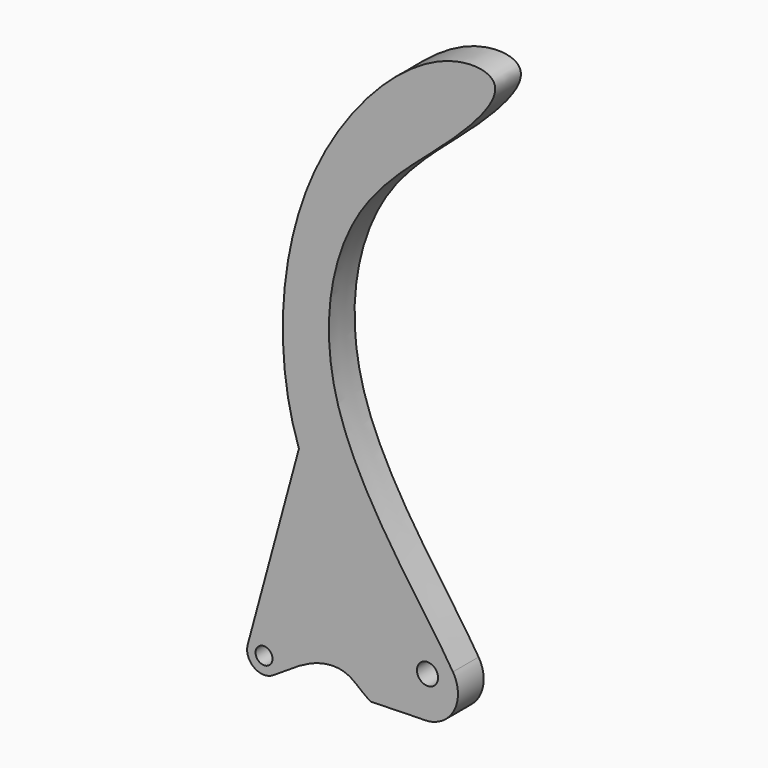
from build123d import *

# Parameters (mm, degrees)
F0_R     = 1.27
F0_R_2   = 1.5875
F1_DEPTH = 4.826
F2_R     = 5.08


with BuildPart() as f1:
    # F0 (on Front) → F1 (new body)
    with BuildSketch(Plane.XZ):
        with BuildLine():
            add(Edge.make_bspline(
                [(-5.7409273062, -27.357215091), (-3.6683374093, -26.0328951082), (-0.0251701264, -23.2850982777), (5.6115406498, -22.8429500303), (7.6257882882, -25.3641492448), (8.9509775862, -26.0758455843)],
                knots=[0, 0, 0, 0, 0.3817939574, 0.6994189819, 1, 1, 1, 1], degree=3))
            Line((8.9509775862, -26.0758455843), (16.1743344595, -25.8907967367))
            add(Edge.make_bspline(
                [(16.1743344595, -25.8907967367), (14.5463270907, -22.5263236355), (12.9183197219, -19.1618505343), (10.2751832414, -15.4096915571)],
                knots=[0, 0, 0, 0, 0.077888926, 0.077888926, 0.077888926, 0.077888926], degree=3))
            add(Edge.make_bspline(
                [(10.2751832414, -15.4096915571), (6.6364516561, -10.2441999209), (1.0738216148, -4.3439561733), (-1.8614867632, 3.8848498313)],
                knots=[0.077888926, 0.077888926, 0.077888926, 0.077888926, 0.1851164178, 0.1851164178, 0.1851164178, 0.1851164178], degree=3))
            Line((-1.8614867632, 3.8848498313), (-9.560300399, -24.553100254))
            ThreePointArc((-9.560300399, -24.553100254), (-6.7737644216, -22.6990049585), (-4.5685573119, -25.216844056))
            ThreePointArc((-4.5685573119, -25.216844056), (-4.8808477017, -26.4370530106), (-5.7409273062, -27.357215091))
        make_face()
        with BuildLine():
            ThreePointArc((-9.560300399, -24.553100254), (-8.6117506787, -27.264283848), (-5.7409273062, -27.357215091))
            ThreePointArc((-5.7409273062, -27.357215091), (-4.8808477017, -26.4370530106), (-4.5685573119, -25.216844056))
            ThreePointArc((-4.5685573119, -25.216844056), (-6.7737644216, -22.6990049585), (-9.560300399, -24.553100254))
        make_face()
        with Locations((-7.1085573119, -25.216844056)):
            Circle(F0_R, mode=Mode.SUBTRACT)
        with BuildLine():
            add(Edge.make_bspline(
                [(16.1743344595, -25.8907967367), (14.5463270907, -22.5263236355), (12.9183197219, -19.1618505343), (10.2751832414, -15.4096915571)],
                knots=[0, 0, 0, 0, 0.077888926, 0.077888926, 0.077888926, 0.077888926], degree=3))
            Line((16.1743344595, -25.8907967367), (25.5930349231, -25.8907967367))
            add(Edge.make_bspline(
                [(-1.8614867632, 3.8848498313), (-5.5713200583, 14.284949093), (-4.6432671747, 41.195895922), (17.1641890949, 64.2564894171), (30.9795358991, 62.8017285805), (20.3263989801, 50.5876190519), (4.3365893948, 39.2173794204), (-0.4864534789, 10.7428135064), (19.8393789476, -14.7354313612), (23.9996070336, -22.8014096788), (25.5930349231, -25.8907967367)],
                knots=[0.1851164178, 0.1851164178, 0.1851164178, 0.1851164178, 0.3206374834, 0.4434091583, 0.50463888, 0.5800628175, 0.6816083979, 0.7958783822, 0.9218184504, 1, 1, 1, 1], degree=3))
            add(Edge.make_bspline(
                [(10.2751832414, -15.4096915571), (6.6364516561, -10.2441999209), (1.0738216148, -4.3439561733), (-1.8614867632, 3.8848498313)],
                knots=[0.077888926, 0.077888926, 0.077888926, 0.077888926, 0.1851164178, 0.1851164178, 0.1851164178, 0.1851164178], degree=3))
        make_face()
        with Locations((17.4575652927, -19.6446664631)):
            Circle(F0_R_2, mode=Mode.SUBTRACT)
    extrude(amount=F1_DEPTH)

    # F2
    f2_edges = [f1.edges().sort_by_distance(p)[0] for p in [
        (16.174334, -2.413, -25.890797),
        (25.593035, -2.413, -25.890797),
    ]]
    fillet(f2_edges, radius=F2_R)


solid = f1.part
